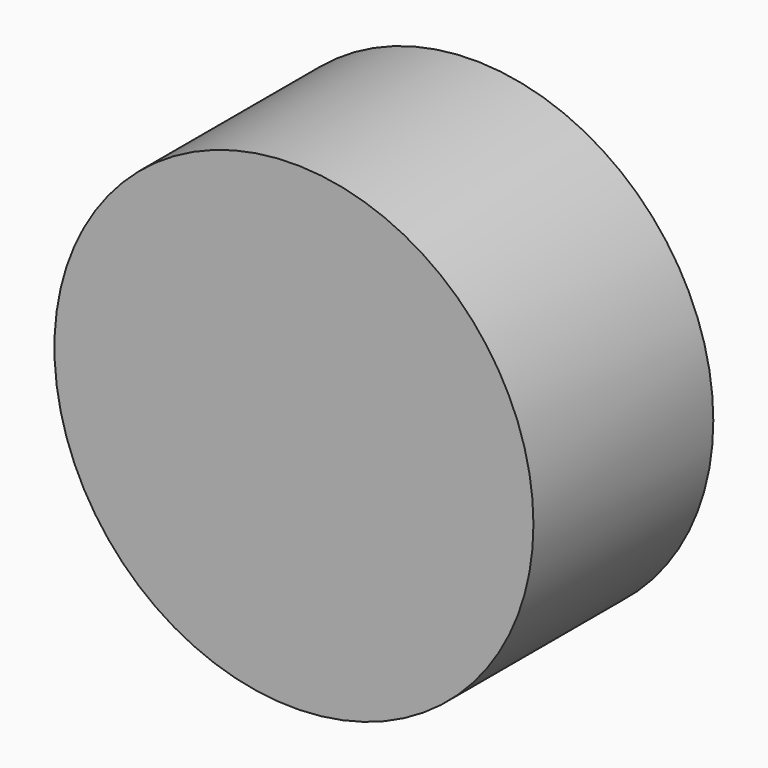
from build123d import *

# Parameters (mm, degrees)
F0_R     = 26.6302362031
F1_DEPTH = 25


# Not quite as in the source:
# - the program builds the solid bodies; features that only make, move or delete a surface that nothing else refers to are left out


with BuildPart() as f1:
    # F0 (on Front) → F1 (new body)
    with BuildSketch(Plane.XZ):
        Circle(F0_R)
    extrude(amount=F1_DEPTH)


solid = f1.part
